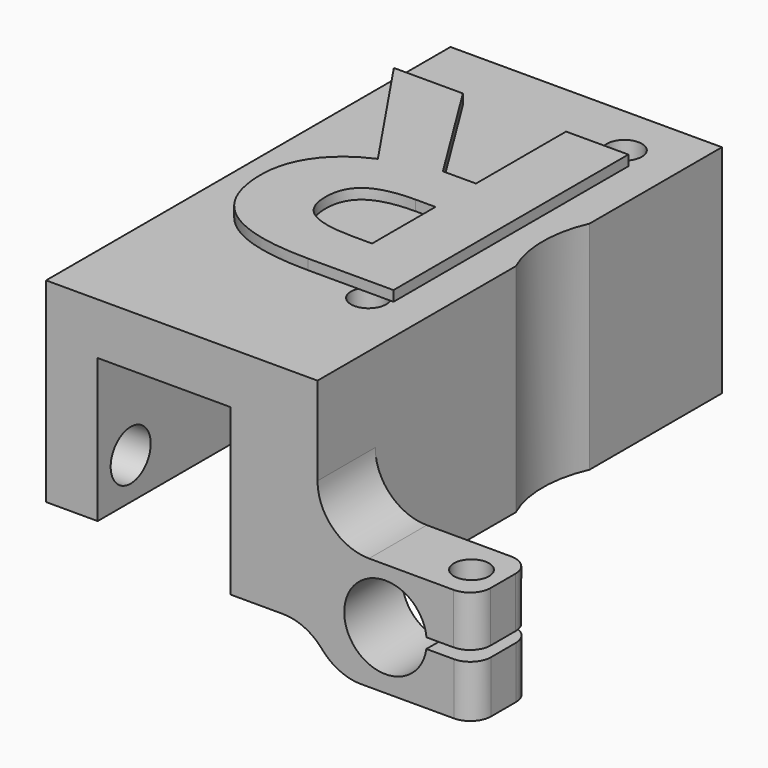
from build123d import *

# Parameters (mm, degrees)
F1_DEPTH      = 7
F2_DEPTH      = 42
F3_R          = 1.7
F3_R_2        = 11
F4_DEPTH      = 21.001
F5_R          = 4
F6_DEPTH      = 10
F7_DEPTH      = 21.001
F8_R          = 1.4
F9_DEPTH      = 11.021861364
F8_R_2        = 1.7
F10_DEPTH     = 4.9110969969
F11_R         = 5
F12_R         = 5
F13_R         = 5
F14_R         = 2
F15_R         = 2.2
F15_R_2       = 2.4255023423
F16_DEPTH     = 6
F17_TEXT_SIZE = 39.8544369641
F18_DEPTH     = 1


# Not quite as in the source:
# - a feature names something its author has since deleted; it is built from what else it names
# - Text() gives the source's letters only with a copy of the font that has no kerning and outlines rounded to 1/6400 em; it was checked with that copy


with BuildPart() as f1:
    # F0 (on Front) → F1 (new body)
    with BuildSketch(Plane.XZ):
        Polygon((-18.6721007523, 29.8099789735), (-18.6721007523, 10.8925135386), (-13.6721007523, 10.8925135386), (-13.6721007523, 24.8099789735), (-0.7721007523, 24.8099789735), (-0.7721007523, 8.8099789735), (7.6380548998, 8.8099789735), (7.6380548998, 16.2656020473), (7.6380548998, 29.8099789735), align=None)
        Polygon((22.8263195603, 16.2417280634), (7.6380548998, 16.2656020473), (7.6380548998, 8.8099789735), (9.0533044869, 5.2860832236), (22.8553367778, 5.2860832236), (22.8553367778, 10.343908232), (16.1860510706, 10.343908232), (16.1860510706, 11.3388913612), (22.8263195603, 11.3388913612), align=None)
    extrude(amount=F1_DEPTH)

    # F0 (on Front) → F2 (join)
    with BuildSketch(Plane.XZ):
        Polygon((-18.6721007523, 29.8099789735), (-18.6721007523, 10.8925135386), (-13.6721007523, 10.8925135386), (-13.6721007523, 24.8099789735), (-0.7721007523, 24.8099789735), (-0.7721007523, 8.8099789735), (7.6380548998, 8.8099789735), (7.6380548998, 16.2656020473), (7.6380548998, 29.8099789735), align=None)
    extrude(amount=-F2_DEPTH)

    # F3 (on face) → F4 (cut, through all)
    with BuildSketch(Plane(origin=(0, 0, 8.8099789735), x_dir=(1, 0, 0), z_dir=(0, 0, -1))):
        with Locations((2.1850741468, -6)):
            Circle(F3_R)
        with Locations((2.1850741468, -37)):
            Circle(F3_R)
        with Locations((17.6850741468, -21.5)):
            Circle(F3_R_2)
    extrude(amount=-F4_DEPTH, mode=Mode.SUBTRACT)

    # F5 (on face) → F6 (cut)
    with BuildSketch(Plane.XZ.offset(7)):
        with Locations((14.2278992477, 10.8989789735)):
            Circle(F5_R)
    extrude(amount=-F6_DEPTH, mode=Mode.SUBTRACT)

    # F3 (on face) → F7 (cut, through all)
    with BuildSketch(Plane(origin=(0, 0, 8.8099789735), x_dir=(1, 0, 0), z_dir=(0, 0, -1))):
        with Locations((2.1850741468, -6)):
            Circle(F3_R)
        with Locations((2.1850741468, -37)):
            Circle(F3_R)
        with Locations((17.6850741468, -21.5)):
            Circle(F3_R_2)
    extrude(amount=-F7_DEPTH, mode=Mode.SUBTRACT)

    # F8 (on face) → F9 (cut, through all)
    with BuildSketch(Plane(origin=(0.0255862274, 0, 16.2775678616), x_dir=(0.9999987646, 0, -0.0015718685), z_dir=(0.0015718685, 0, 0.9999987646))):
        with Locations((19.8007615007, -3.5767070949)):
            Circle(F8_R)
    extrude(amount=-F9_DEPTH, mode=Mode.SUBTRACT)

    # F8 (on face) → F10 (cut, through all)
    with BuildSketch(Plane(origin=(0.0255862274, 0, 16.2775678616), x_dir=(0.9999987646, 0, -0.0015718685), z_dir=(0.0015718685, 0, 0.9999987646))):
        with Locations((19.8007615007, -3.5767070949)):
            Circle(F8_R_2)
        with Locations((19.8007615007, -3.5767070949)):
            Circle(F8_R, mode=Mode.SUBTRACT)
    extrude(amount=-F10_DEPTH, mode=Mode.SUBTRACT)

    # F11
    f11_edges = [f1.edges().sort_by_distance(p)[0] for p in [
        (7.638055, -3.5, 16.265602),
    ]]
    fillet(f11_edges, radius=F11_R)

    # F12
    f12_edges = [f1.edges().sort_by_distance(p)[0] for p in [
        (7.638055, -3.5, 8.809979),
    ]]
    fillet(f12_edges, radius=F12_R)

    # F13
    f13_edges = [f1.edges().sort_by_distance(p)[0] for p in [
        (9.053304, -3.5, 5.286083),
    ]]
    fillet(f13_edges, radius=F13_R)

    # F14
    f14_edges = [f1.edges().sort_by_distance(p)[0] for p in [
        (22.82632, -7, 13.79031),
        (22.855337, -7, 7.814996),
        (22.82632, 0, 13.79031),
        (22.855337, 0, 7.814996),
    ]]
    fillet(f14_edges, radius=F14_R)

    # F15 (on face) → F16 (cut)
    with BuildSketch(Plane(origin=(-18.6721007523, 0, 0), x_dir=(0, -1, 0), z_dir=(-1, 0, 0))):
        with Locations((-38, 14.8925135386)):
            Circle(F15_R)
        with Locations((3, 14.8925135386)):
            Circle(F15_R_2)
    extrude(amount=-F16_DEPTH, mode=Mode.SUBTRACT)

    # F17 (on face) → F18 (join)
    with BuildSketch(Plane.XY.offset(29.8099789735)):
        with Locations(Location((7.6380548998, 35.1361208781), (0, 0, 180))):
            Text('R', F17_TEXT_SIZE, font='Open Sans', font_style=FontStyle.BOLD, text_align=(TextAlign.LEFT, TextAlign.BOTTOM))
    extrude(amount=F18_DEPTH)


solid = f1.part
